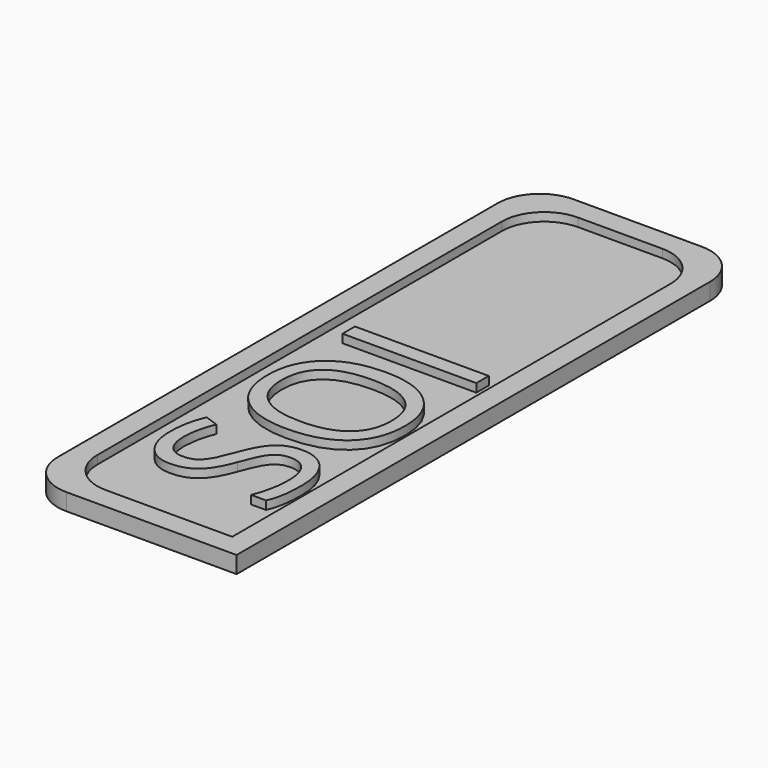
from build123d import *

# Parameters (mm, degrees)
F0_TEXT_SIZE = 28.2222222222
F1_DEPTH     = 2.54
F3_DEPTH     = 1.27


# Not quite as in the source:
# - Text() gives the source's letters only with a copy of the font that has no kerning and outlines rounded to 1/6400 em; it was checked with that copy


with BuildPart() as f1:
    # F0 (on Top) → F1 (new body)
    with BuildSketch(Plane.XY):
        with BuildLine():
            ThreePointArc((-9.6519991798, 43.4968434274), (-14.1421272404, 41.636971488), (-16.0019991798, 37.1468434274))
            Line((-16.0019991798, 37.1468434274), (-16.0019991798, -45.6571549323))
            ThreePointArc((-16.0019991798, -45.6571549323), (-14.1421272404, -50.1472829928), (-9.6519991798, -52.0071549323))
            Line((-9.6519991798, -52.0071549323), (0, -52.0071549323))
            Line((0, -52.0071549323), (16.0019991798, -52.0071549323))
            Line((16.0019991798, -52.0071549323), (16.0019991798, 37.1468434274))
            ThreePointArc((16.0019991798, 37.1468434274), (14.1421272404, 41.636971488), (9.6519991798, 43.4968434274))
            Line((9.6519991798, 43.4968434274), (0, 43.4968434274))
            Line((0, 43.4968434274), (-9.6519991798, 43.4968434274))
        make_face()
        with BuildLine():
            ThreePointArc((-12.7, 33.8448442476), (-10.8401280605, 38.3349723081), (-6.35, 40.1948442476))
            Line((-6.35, 40.1948442476), (0, 40.1948442476))
            Line((0, 40.1948442476), (6.35, 40.1948442476))
            ThreePointArc((6.35, 40.1948442476), (10.8401280605, 38.3349723081), (12.7, 33.8448442476))
            Line((12.7, 33.8448442476), (12.7, -48.7051557524))
            Line((12.7, -48.7051557524), (0, -48.7051557524))
            Line((0, -48.7051557524), (-6.35, -48.7051557524))
            ThreePointArc((-6.35, -48.7051557524), (-10.8401280605, -46.845283813), (-12.7, -42.3551557524))
            Line((-12.7, -42.3551557524), (-12.7, 33.8448442476))
        make_face(mode=Mode.SUBTRACT)
        with Locations(Location((10.6680010107, -40.4468369429), (0, 0, 90))):
            Text('SOI', F0_TEXT_SIZE, font='Open Sans', text_align=(TextAlign.LEFT, TextAlign.BOTTOM))
    extrude(amount=F1_DEPTH)


with BuildPart() as f3:
    # F2 (on Top) → F3 (new body)
    with BuildSketch(Plane.XY):
        with BuildLine():
            Line((-0.0242226921, 40.272474432), (-6.3742226921, 40.272474432))
            ThreePointArc((-6.3742226921, 40.272474432), (-10.8643507526, 38.4126024925), (-12.7242226921, 33.922474432))
            Line((-12.7242226921, 33.922474432), (-12.7242226921, -42.277525568))
            ThreePointArc((-12.7242226921, -42.277525568), (-10.8643507526, -46.7676536285), (-6.3742226921, -48.627525568))
            Line((-6.3742226921, -48.627525568), (-0.0242226921, -48.627525568))
            Line((-0.0242226921, -48.627525568), (12.6757773079, -48.627525568))
            Line((12.6757773079, -48.627525568), (12.6757773079, 33.922474432))
            ThreePointArc((12.6757773079, 33.922474432), (10.8159053684, 38.4126024925), (6.3257773079, 40.272474432))
            Line((6.3257773079, 40.272474432), (-0.0242226921, 40.272474432))
        make_face()
    extrude(amount=F3_DEPTH)


solid = Compound([f1.part, f3.part])
